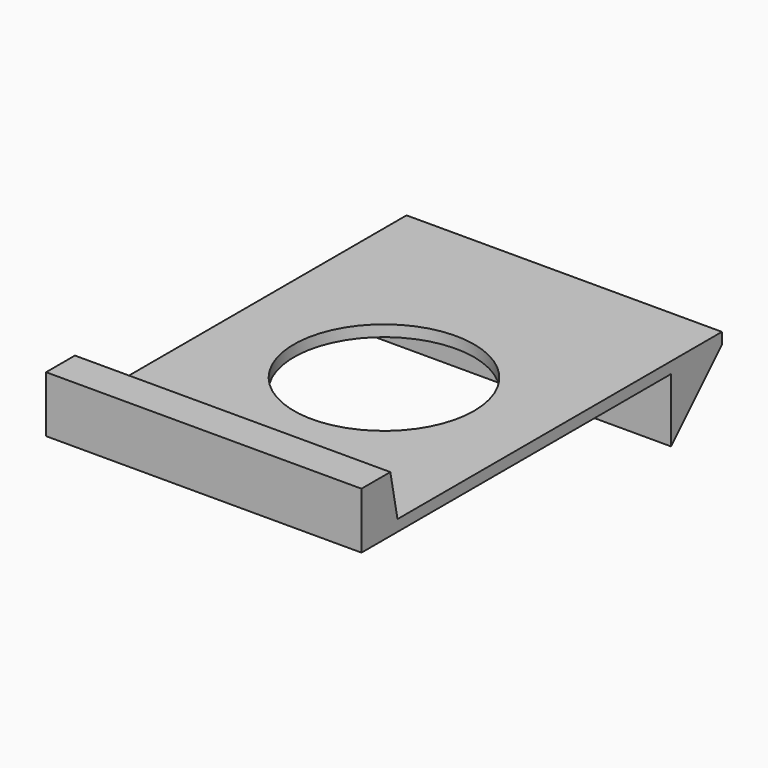
from build123d import *

# Parameters (mm, degrees)
F0_W     = 88.9
F0_H     = 127
F1_DEPTH = 3.175
F2_W     = 88.9
F2_H     = 17.9578
F3_DEPTH = 17.9578
F4_SIZE  = 17.95779
F5_R     = 25.4
F6_DEPTH = 3.175
F7_W     = 88.9
F7_H     = 12.7
F8_DEPTH = 12.7
F9_SIZE2 = 12.69999
F9_SIZE  = 2.53999


# Not quite as in the source:
# - a fillet or chamfer is up to 0.001 mm smaller than in the source, because OpenCascade refuses the exact size


with BuildPart() as f1:
    # F0 (on Top) → F1 (new body)
    with BuildSketch(Plane.XY):
        Rectangle(F0_W, F0_H)
    extrude(amount=F1_DEPTH)

    # F2 (on face) → F3 (join)
    with BuildSketch(Plane(origin=(0, 0, 0), x_dir=(1, 0, 0), z_dir=(0, 0, -1))):
        with Locations((0, -54.5211)):
            Rectangle(F2_W, F2_H)
    extrude(amount=F3_DEPTH)

    # F4 (size 17.9578 in the source; OpenCascade refuses exactly that, so slightly less here)
    f4_edges = [f1.edges().sort_by_distance(p)[0] for p in [
        (0, 63.5, -17.9578),
    ]]
    chamfer(f4_edges, length=F4_SIZE)

    # F5 (on face) → F6 (cut)
    with BuildSketch(Plane.XY.offset(3.175)):
        Circle(F5_R)
    extrude(amount=-F6_DEPTH, mode=Mode.SUBTRACT)

    # F7 (on face) → F8 (join)
    with BuildSketch(Plane.XY.offset(3.175)):
        with Locations((0, -57.15)):
            Rectangle(F7_W, F7_H)
    extrude(amount=F8_DEPTH)

    # F9 (size 2.54 and 12.7 in the source; OpenCascade refuses exactly that, so slightly less here)
    f9_edges = [f1.edges().sort_by_distance(p)[0] for p in [
        (0, -50.8, 15.875),
    ]]
    f9_side = f1.faces().sort_by_distance((0, -57.15, 15.875))[0]
    chamfer(f9_edges, length=F9_SIZE, length2=F9_SIZE2, reference=f9_side)


solid = f1.part
